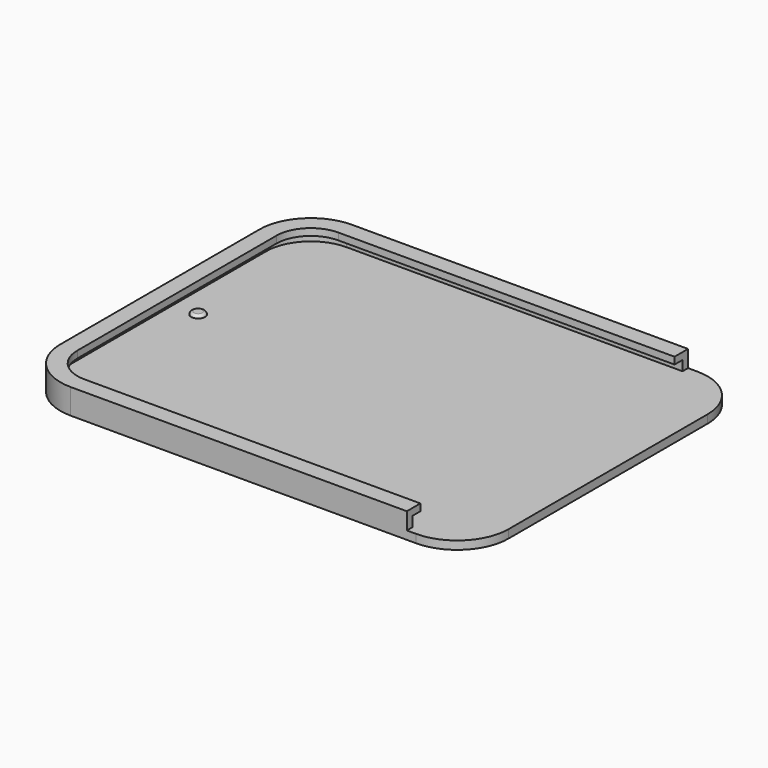
from build123d import *

# Parameters (mm, degrees)
F1_DEPTH = 3.65
F3_DEPTH = 2.45
F5_DEPTH = 1
F6_W     = 11.5363439545
F6_H     = 60.74937433
F7_DEPTH = 25
F8_R     = 1
F9_DEPTH = 0.4
F10_R    = 0.39999


# Not quite as in the source:
# - a fillet or chamfer is up to 0.001 mm smaller than in the source, because OpenCascade refuses the exact size


with BuildPart() as f1:
    # F0 (on Top) → F1 (new body)
    with BuildSketch(Plane.XY):
        with BuildLine():
            ThreePointArc((-62.0253431911, -15.11933375), (-59.843288711, -20.3872792698), (-54.5753431911, -22.56933375))
            Line((-54.5753431911, -22.56933375), (-4.5753431911, -22.56933375))
            ThreePointArc((-4.5753431911, -22.56933375), (0.6926023287, -20.3872792698), (2.8746568089, -15.11933375))
            Line((2.8746568089, -15.11933375), (2.8746568089, 20.88066625))
            ThreePointArc((2.8746568089, 20.88066625), (0.6926023287, 26.1486117698), (-4.5753431911, 28.33066625))
            Line((-4.5753431911, 28.33066625), (-54.5753431911, 28.33066625))
            ThreePointArc((-54.5753431911, 28.33066625), (-59.843288711, 26.1486117698), (-62.0253431911, 20.88066625))
            Line((-62.0253431911, 20.88066625), (-62.0253431911, -15.11933375))
        make_face()
    extrude(amount=F1_DEPTH)

    # F2 (on face) → F3 (cut)
    with BuildSketch(Plane.XY.offset(3.65)):
        with BuildLine():
            Line((1.8746568089, -15.11933375), (1.8746568089, 20.88066625))
            ThreePointArc((1.8746568089, 20.88066625), (-0.0145044525, 25.4415049886), (-4.5753431911, 27.33066625))
            Line((-4.5753431911, 27.33066625), (-54.5753431911, 27.33066625))
            ThreePointArc((-54.5753431911, 27.33066625), (-59.1361819298, 25.4415049886), (-61.0253431911, 20.88066625))
            Line((-61.0253431911, 20.88066625), (-61.0253431911, -15.11933375))
            ThreePointArc((-61.0253431911, -15.11933375), (-59.1361819298, -19.6801724887), (-54.5753431911, -21.56933375))
            Line((-54.5753431911, -21.56933375), (-4.5753431911, -21.56933375))
            ThreePointArc((-4.5753431911, -21.56933375), (-0.0145044525, -19.6801724887), (1.8746568089, -15.11933375))
        make_face()
    extrude(amount=-F3_DEPTH, mode=Mode.SUBTRACT)

    # F4 (on face) → F5 (join)
    with BuildSketch(Plane.XY.offset(3.65)):
        with BuildLine():
            Line((1.8746568089, -15.11933375), (1.8746568089, 20.88066625))
            ThreePointArc((1.8746568089, 20.88066625), (-0.0145044525, 25.4415049886), (-4.5753431911, 27.33066625))
            Line((-4.5753431911, 27.33066625), (-54.5753431911, 27.33066625))
            ThreePointArc((-54.5753431911, 27.33066625), (-59.1361819298, 25.4415049886), (-61.0253431911, 20.88066625))
            Line((-61.0253431911, 20.88066625), (-61.0253431911, -15.11933375))
            ThreePointArc((-61.0253431911, -15.11933375), (-59.1361819298, -19.6801724887), (-54.5753431911, -21.56933375))
            Line((-54.5753431911, -21.56933375), (-4.5753431911, -21.56933375))
            ThreePointArc((-4.5753431911, -21.56933375), (-0.0145044525, -19.6801724887), (1.8746568089, -15.11933375))
        make_face()
        with BuildLine():
            ThreePointArc((-4.5753431911, 25.88066625), (-1.0398092852, 24.4162001559), (0.4246568089, 20.88066625))
            Line((0.4246568089, 20.88066625), (0.4246568089, -15.11933375))
            ThreePointArc((0.4246568089, -15.11933375), (-1.0398092852, -18.6548676559), (-4.5753431911, -20.11933375))
            Line((-4.5753431911, -20.11933375), (-54.5753431911, -20.11933375))
            ThreePointArc((-54.5753431911, -20.11933375), (-58.1108770971, -18.6548676559), (-59.5753431911, -15.11933375))
            Line((-59.5753431911, -15.11933375), (-59.5753431911, 20.88066625))
            ThreePointArc((-59.5753431911, 20.88066625), (-58.1108770971, 24.4162001559), (-54.5753431911, 25.88066625))
            Line((-54.5753431911, 25.88066625), (-4.5753431911, 25.88066625))
        make_face(mode=Mode.SUBTRACT)
    extrude(amount=-F5_DEPTH)

    # F6 (on face) → F7 (cut)
    with BuildSketch(Plane.XY.offset(1.2)):
        with Locations((-0.1405403018, 2.3494064808)):
            Rectangle(F6_W, F6_H)
    extrude(amount=F7_DEPTH, mode=Mode.SUBTRACT)

    # F8 (on face) → F9 (join)
    with BuildSketch(Plane.XY.offset(1.2)):
        with Locations((-57.3753431911, 3.9823222905)):
            Circle(F8_R)
    extrude(amount=F9_DEPTH)

    # F10 (radius 0.4 in the source; OpenCascade refuses exactly that, so slightly less here)
    f10_edges = [f1.edges().sort_by_distance(p)[0] for p in [
        (-58.375343, 3.982322, 1.6),
    ]]
    fillet(f10_edges, radius=F10_R)


solid = f1.part
